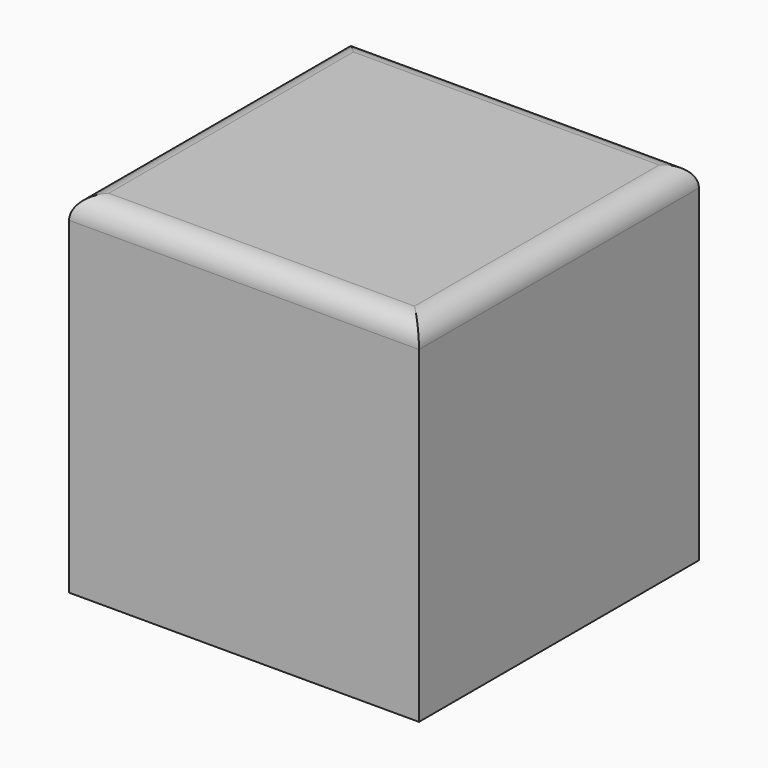
from build123d import *

# Parameters (mm, degrees)
F0_W     = 127
F0_H     = 127
F1_DEPTH = 63.5
F2_R     = 8


# Not quite as in the source:
# - the program builds the solid bodies; features that only make, move or delete a surface that nothing else refers to are left out


with BuildPart() as f1:
    # F0 (on Front) → F1 (new body, symmetric)
    with BuildSketch(Plane.XZ):
        Rectangle(F0_W, F0_H)
    extrude(amount=F1_DEPTH, both=True)

    # F2
    f2_edges = [f1.edges().sort_by_distance(p)[0] for p in [
        (63.5, 0, 63.5),
        (0, 63.5, 63.5),
        (-63.5, 0, 63.5),
        (0, -63.5, 63.5),
    ]]
    fillet(f2_edges, radius=F2_R)


solid = f1.part
